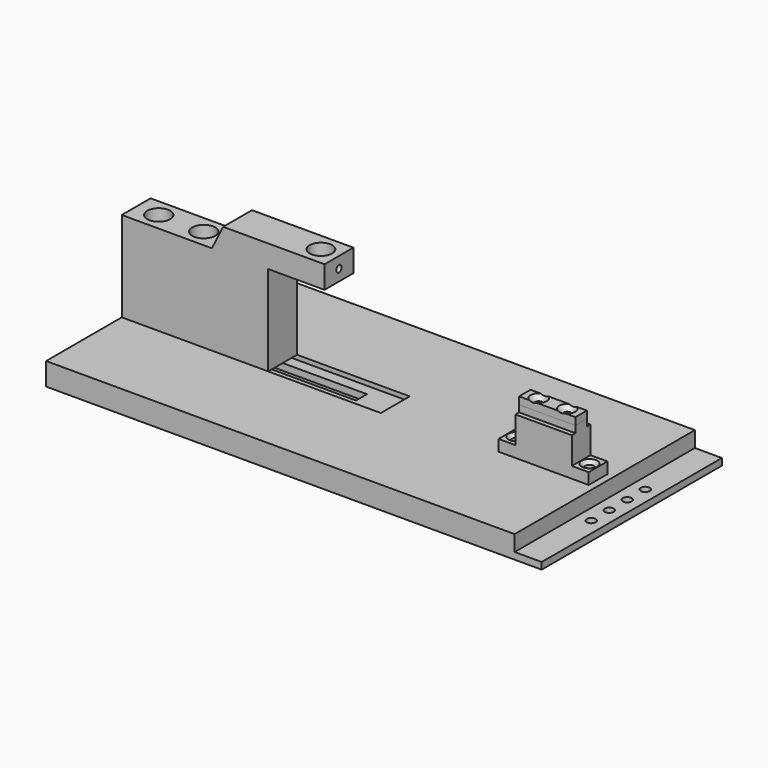
from build123d import *

# Parameters (mm, degrees)
F0_W      = 220
F0_H      = 100
F1_DEPTH  = 10
F2_W      = 40
F2_H      = 10.35
F2_R      = 2
F3_DEPTH  = 20
F4_W      = 7.5
F4_H      = 15
F5_DEPTH  = 55.176
F6_R      = 1.5
F7_DEPTH  = 10
F8_W      = 25
F8_H      = 2
F9_DEPTH  = 3
F10_SIZE  = 1.5
F11_R     = 2
F12_DEPTH = 10.001
F13_W     = 25
F13_H     = 6.35
F13_R     = 1.6
F14_DEPTH = 3.25
F16_W     = 100
F16_H     = 6.1
F17_DEPTH = 25
F18_W     = 100
F18_H     = 10.5
F19_DEPTH = 5
F20_R     = 2
F21_DEPTH = 10.001
F24_DEPTH = 8
F25_R     = 3.05
F26_DEPTH = 40
F27_R     = 5.1
F28_DEPTH = 6.1
F29_R     = 5
F30_DEPTH = 10
F31_R     = 1.5
F32_DEPTH = 3.2313040929
F33_W     = 12
F33_H     = 100
F34_DEPTH = 7
F35_W     = 115
F35_H     = 16
F36_DEPTH = 2


# Not quite as in the source:
# - a fillet or chamfer that OpenCascade refuses, or shapes differently, is made with other operations: its cross-section is extruded or revolved along the edge and cut away or added


with BuildPart() as f1:
    # F0 (on Top) → F1 (new body)
    with BuildSketch(Plane.XY):
        with Locations((110, 50)):
            Rectangle(F0_W, F0_H)
    extrude(amount=F1_DEPTH)

    # F11 (on face) → F12 (cut, through all)
    with BuildSketch(Plane.XY.offset(10)):
        with Locations((168.75, 50)):
            Circle(F11_R)
        with Locations((201.25, 50)):
            Circle(F11_R)
        with Locations((214, 65)):
            Circle(F11_R)
        with Locations((214, 55)):
            Circle(F11_R)
        with Locations((214, 45)):
            Circle(F11_R)
        with Locations((214, 35)):
            Circle(F11_R)
    extrude(amount=-F12_DEPTH, mode=Mode.SUBTRACT)

    # F16 (on face) → F17 (cut)
    with BuildSketch(Plane(origin=(0, 0, 0), x_dir=(1, 0, 0), z_dir=(0, 0, -1))):
        with Locations((50, -50)):
            Rectangle(F16_W, F16_H)
    extrude(amount=-F17_DEPTH, mode=Mode.SUBTRACT)

    # F18 (on face) → F19 (cut)
    with BuildSketch(Plane(origin=(0, 0, 0), x_dir=(1, 0, 0), z_dir=(0, 0, -1))):
        with Locations((50, -50)):
            Rectangle(F18_W, F18_H)
    extrude(amount=-F19_DEPTH, mode=Mode.SUBTRACT)

    # F20 (on face) → F21 (cut, through all)
    with BuildSketch(Plane.XY.offset(10)):
        with Locations((168.75, 50)):
            Circle(F20_R)
        with Locations((201.25, 50)):
            Circle(F20_R)
    extrude(amount=-F21_DEPTH, mode=Mode.SUBTRACT)

    # F33 (on face) → F34 (cut)
    with BuildSketch(Plane.XY.offset(10)):
        with Locations((214, 50)):
            Rectangle(F33_W, F33_H)
    extrude(amount=-F34_DEPTH, mode=Mode.SUBTRACT)

    # F35 (on face) → F36 (cut)
    with BuildSketch(Plane.XY.offset(10)):
        with Locations((57.5, 50)):
            Rectangle(F35_W, F35_H)
    extrude(amount=-F36_DEPTH, mode=Mode.SUBTRACT)


with BuildPart() as f3:
    # F2 (on face) → F3 (new body)
    with BuildSketch(Plane.XY.offset(10)):
        with Locations((185, 50)):
            Rectangle(F2_W, F2_H)
        with Locations((168.75, 50)):
            Circle(F2_R, mode=Mode.SUBTRACT)
        with Locations((201.25, 50)):
            Circle(F2_R, mode=Mode.SUBTRACT)
    extrude(amount=F3_DEPTH)

    # F4 (on face) → F5 (cut, through all)
    with BuildSketch(Plane.XZ.offset(-44.825)):
        with Locations((168.75, 22.5)):
            Rectangle(F4_W, F4_H)
        with Locations((201.25, 22.5)):
            Rectangle(F4_W, F4_H)
    extrude(amount=-F5_DEPTH, mode=Mode.SUBTRACT)

    # F6 (on face) → F7 (cut)
    with BuildSketch(Plane.XY.offset(30)):
        with Locations((178.65, 50)):
            Circle(F6_R)
        with Locations((191.35, 50)):
            Circle(F6_R)
    extrude(amount=-F7_DEPTH, mode=Mode.SUBTRACT)

    # F8 (on face) → F9 (cut)
    with BuildSketch(Plane.XY.offset(30)):
        with Locations((185, 54.175)):
            Rectangle(F8_W, F8_H)
        with Locations((185, 45.825)):
            Rectangle(F8_W, F8_H)
    extrude(amount=-F9_DEPTH, mode=Mode.SUBTRACT)

    # F10
    f10_edges = [f3.edges().sort_by_distance(p)[0] for p in [
        (166.75, 50, 15),
        (199.25, 50, 15),
    ]]
    chamfer(f10_edges, length=F10_SIZE)


with BuildPart() as f14:
    # F13 (on face) → F14 (new body)
    with BuildSketch(Plane.XY.offset(30)):
        with Locations((185, 50)):
            Rectangle(F13_W, F13_H)
        with Locations((178.65, 50)):
            Circle(F13_R, mode=Mode.SUBTRACT)
        with Locations((191.35, 50)):
            Circle(F13_R, mode=Mode.SUBTRACT)
    extrude(amount=F14_DEPTH)

    # F15: chamfer of 2 on 2 edges, made by hand

    # F15_s1 → F15_t2 (revolve, cut)
    with BuildSketch(Plane.XZ.offset(-50)):
        Polygon((180.25, 31.25), (182.25, 33.25), (180.25, 33.25), align=None)
    revolve(axis=Axis((178.65, 50, 33.25), (0, 0, 1)), mode=Mode.SUBTRACT)

    # F15_s3 → F15_t4 (revolve, cut)
    with BuildSketch(Plane.XZ.offset(-50)):
        Polygon((192.95, 31.25), (194.95, 33.25), (192.95, 33.25), align=None)
    revolve(axis=Axis((191.35, 50, 33.25), (0, 0, 1)), mode=Mode.SUBTRACT)


with BuildPart() as f24:
    # F23 (on offset) → F24 (new body, symmetric)
    with BuildSketch(Plane.XZ.offset(-50)):
        Polygon((0, 50), (0, 10), (65, 10), (65, 50), (90, 50), (90, 60), (45, 60), (40, 50), align=None)
    extrude(amount=F24_DEPTH, both=True)

    # F25 (on face) → F26 (cut, through all)
    with BuildSketch(Plane.XY.offset(50)):
        with Locations((10, 50)):
            Circle(F25_R)
        with Locations((30, 50)):
            Circle(F25_R)
    extrude(amount=-F26_DEPTH, mode=Mode.SUBTRACT)

    # F27 (on face) → F28 (cut)
    with BuildSketch(Plane.XY.offset(50)):
        with Locations((10, 50)):
            Circle(F27_R)
        with Locations((30, 50)):
            Circle(F27_R)
    extrude(amount=-F28_DEPTH, mode=Mode.SUBTRACT)

    # F29 (on face) → F30 (cut, through all)
    with BuildSketch(Plane.XY.offset(60)):
        with Locations((82, 50)):
            Circle(F29_R)
    extrude(amount=-F30_DEPTH, mode=Mode.SUBTRACT)

    # F31 (on face) → F32 (cut, through all)
    with BuildSketch(Plane.YZ.offset(90)):
        with Locations((50, 55)):
            Circle(F31_R)
    extrude(amount=-F32_DEPTH, mode=Mode.SUBTRACT)


solid = Compound([f1.part, f3.part, f14.part, f24.part])
